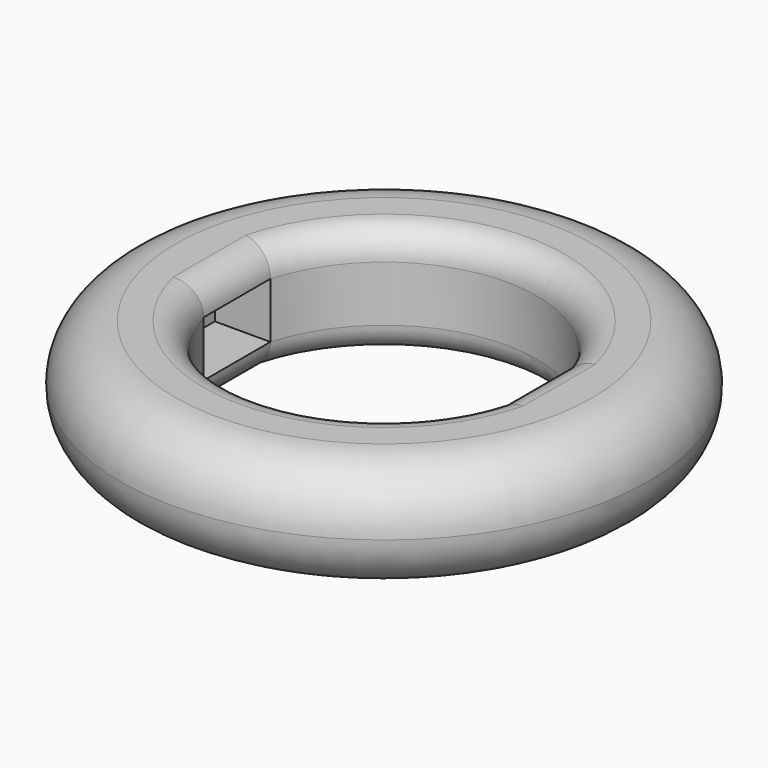
from build123d import *

# Parameters (mm, degrees)
F0_R     = 4.75
F1_DEPTH = 2
F2_W     = 1
F2_H     = 0.5
F3_W     = 1
F3_H     = 0.5
F4_DEPTH = 2.5
F5_R     = 0.49999
F6_R     = 0.99999


# Not quite as in the source:
# - a fillet or chamfer is up to 0.001 mm smaller than in the source, because OpenCascade refuses the exact size


with BuildPart() as f1:
    # F0 (on Top) → F1 (new body)
    with BuildSketch(Plane.XY):
        Circle(F0_R)
        with BuildLine():
            ThreePointArc((-2.6457513111, 0.75), (0, 2.75), (2.6457513111, 0.75))
            Line((2.6457513111, 0.75), (3.6457513111, 0.75))
            Line((3.6457513111, 0.75), (3.6457513111, -0.75))
            Line((3.6457513111, -0.75), (2.6457513111, -0.75))
            ThreePointArc((2.6457513111, -0.75), (0, -2.75), (-2.6457513111, -0.75))
            Line((-2.6457513111, -0.75), (-3.6457513111, -0.75))
            Line((-3.6457513111, -0.75), (-3.6457513111, 0.75))
            Line((-3.6457513111, 0.75), (-2.6457513111, 0.75))
        make_face(mode=Mode.SUBTRACT)
    extrude(amount=F1_DEPTH)

    # F2 (on face) + F3 (on face) → F4 (join)
    with BuildSketch(Plane.XZ.offset(-0.75)):
        with Locations((-3.1457513111, 1.75)):
            Rectangle(F2_W, F2_H)
        with Locations((-3.1457513111, 0.25)):
            Rectangle(F2_W, F2_H)
    with BuildSketch(Plane.XZ.offset(-0.75)):
        with Locations((3.1457513111, 0.25)):
            Rectangle(F3_W, F3_H)
        with Locations((3.1457513111, 1.75)):
            Rectangle(F3_W, F3_H)
    extrude(amount=F4_DEPTH)

    # F5 (radius 0.5 in the source; OpenCascade refuses exactly that, so slightly less here)
    f5_edges = [f1.edges().sort_by_distance(p)[0] for p in [
        (-2.645751, 0, 2),
        (2.645751, 0, 2),
        (0, 2.75, 2),
        (0, -2.75, 2),
        (0, 2.75, 0),
        (0, -2.75, 0),
        (-2.645751, 0, 0),
        (2.645751, 0, 0),
    ]]
    fillet(f5_edges, radius=F5_R)

    # F6 (radius 1 in the source; OpenCascade refuses exactly that, so slightly less here)
    f6_edges = [f1.edges().sort_by_distance(p)[0] for p in [
        (-4.75, 0, 2),
        (-4.75, 0, 0),
    ]]
    fillet(f6_edges, radius=F6_R)


solid = f1.part
